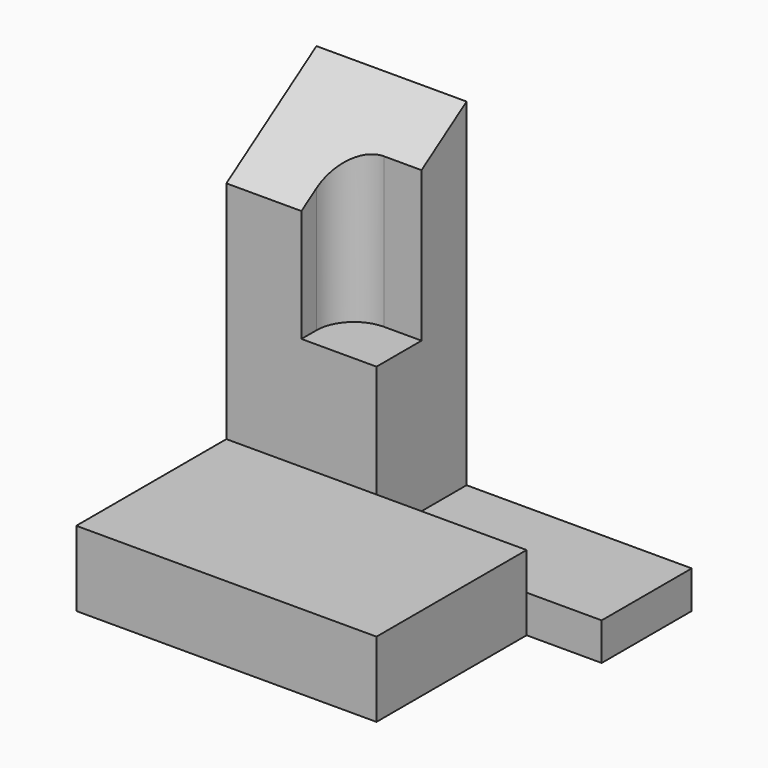
from build123d import *

# Parameters (mm, degrees)
F0_W     = 80
F0_H     = 50
F1_DEPTH = 20
F2_W     = 100
F2_H     = 30
F3_DEPTH = 10
F4_W     = 40
F4_H     = 30
F5_DEPTH = 90
F6_SIZE2 = 19.99999
F6_SIZE  = 29.99999
F9_DEPTH = 50.001


# Not quite as in the source:
# - a fillet or chamfer is up to 0.001 mm smaller than in the source, because OpenCascade refuses the exact size


with BuildPart() as f1:
    # F0 (on Top) → F1 (new body)
    with BuildSketch(Plane.XY):
        with Locations((40, 25)):
            Rectangle(F0_W, F0_H)
    extrude(amount=F1_DEPTH)

    # F2 (on Top) → F3 (join)
    with BuildSketch(Plane.XY):
        with Locations((50, 65)):
            Rectangle(F2_W, F2_H)
    extrude(amount=F3_DEPTH)

    # F4 (on face) → F5 (join)
    with BuildSketch(Plane.XY.offset(10)):
        with Locations((20, 65)):
            Rectangle(F4_W, F4_H)
    extrude(amount=F5_DEPTH)

    # F6 (size 30 and 20 in the source; OpenCascade refuses exactly that, so slightly less here)
    f6_edges = [f1.edges().sort_by_distance(p)[0] for p in [
        (20, 50, 100),
    ]]
    f6_side = f1.faces().sort_by_distance((20, 65, 100))[0]
    chamfer(f6_edges, length=F6_SIZE, length2=F6_SIZE2, reference=f6_side)

    # F8 (on offset) → F9 (cut, through all)
    with BuildSketch(Plane(origin=(0, 0, 50), x_dir=(1, 0, 0), z_dir=(0, 0, -1))):
        with BuildLine():
            Line((30, -65), (40, -65))
            Line((40, -65), (40, -50))
            Line((40, -50), (20, -50))
            Line((20, -50), (20, -55))
            ThreePointArc((20, -55), (22.9289321881, -62.0710678119), (30, -65))
        make_face()
    extrude(amount=-F9_DEPTH, mode=Mode.SUBTRACT)


solid = f1.part
